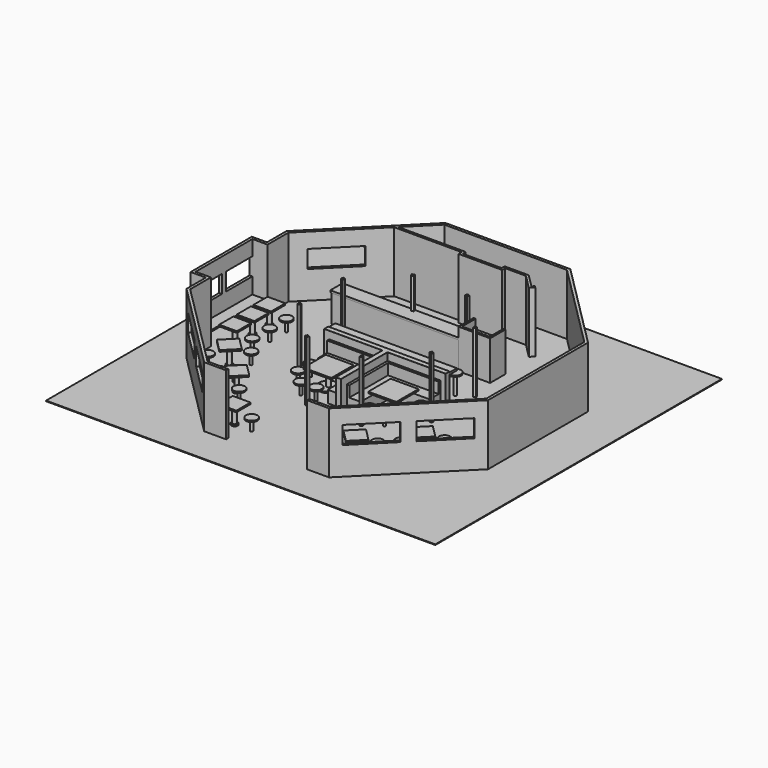
from build123d import *

# Parameters (mm, degrees)
F6_W      = 200
F6_H      = 200
F7_DEPTH  = 1200
F9_DEPTH  = 900
F11_DEPTH = 470
F13_DEPTH = 60
F15_DEPTH = 2400
F17_DEPTH = 2400
F16_W     = 110
F16_H     = 200
F19_W     = 5059.252981
F19_H     = 600
F20_DEPTH = 80
F22_DEPTH = 1550
F23_R     = 3
F25_DEPTH = 80
F27_W     = 110
F27_H     = 1300
F28_DEPTH = 600
F29_W     = 110
F29_H     = 1300
F30_DEPTH = 1100
F31_W     = 5019.252981
F31_H     = 560
F32_DEPTH = 1120
F34_DEPTH = 50
F33_R     = 225
F36_R     = 225
F37_DEPTH = 50
F38_R     = 50
F39_DEPTH = 450
F40_R     = 50
F41_DEPTH = 780
F42_R     = 125
F43_DEPTH = 50
F42_R_2   = 75
F44_R     = 75
F45_DEPTH = 680
F46_R     = 375
F47_DEPTH = 50
F48_R     = 75
F49_DEPTH = 620
F50_W     = 15369.4958686829
F50_H     = 14148.3583450317
F51_DEPTH = 25


# Not quite as in the source:
# - ends of sketch curves that miss each other by under 0.0002 mm in the source are joined


with BuildPart() as f7:
    # F6 (on offset) → F7 (new body)
    with BuildSketch(Plane.XY.offset(1200)):
        Polygon((-108.954118, -103.028913), (-108.954118, 96.971087), (-2306.968571, 96.971087), (-2408.954118, 96.971087), (-2408.954118, -103.028913), (-2208.968571, -103.028913), align=None)
        with Locations((-8.954118, -3.028913)):
            Rectangle(F6_W, F6_H)
        Polygon((91.045882, -103.028913), (-108.954118, -103.028913), (-108.954118, -2112.146564), (-108.954118, -2400), (91.045882, -2400), (91.045882, -2112.146564), align=None)
        Polygon((2289.060335, 96.971087), (91.045882, 96.971087), (91.045882, -103.028913), (2191.060335, -103.028913), (2391.045882, -103.028913), (2391.045882, 96.971087), align=None)
    extrude(amount=-F7_DEPTH)

    # F8 (on offset) → F9 (join)
    with BuildSketch(Plane.XY.offset(900)):
        Polygon((-108.954118, -2112.146564), (-108.954118, -103.028913), (-2208.968571, -103.028913), (-2208.968571, -203.028913), (-208.954118, -203.028913), (-208.954118, -2112.146564), align=None)
        Polygon((91.045882, -103.028913), (91.045882, -2112.146564), (191.045882, -2112.146564), (191.045882, -203.028913), (2191.060335, -203.028913), (2191.060335, -103.028913), align=None)
    extrude(amount=-F9_DEPTH)

    # F10 (on offset) → F11 (join)
    with BuildSketch(Plane.XY.offset(470)):
        Polygon((-2208.968571, -653.028913), (-658.954118, -653.028913), (-658.954118, -2112.146564), (-208.954118, -2112.146564), (-208.954118, -203.028913), (-2208.968571, -203.028913), align=None)
        Polygon((641.045882, -653.028913), (2191.060335, -653.028913), (2191.060335, -203.028913), (191.045882, -203.028913), (191.045882, -2112.146564), (641.045882, -2112.146564), align=None)
    extrude(amount=-F11_DEPTH)

    # F23
    f23_edges = [f7.edges().sort_by_distance(p)[0] for p in [
        (-2408.954118, -3.028913, 1200),
        (-1258.954118, -103.028913, 1200),
        (-108.954118, -1251.514457, 1200),
        (-8.954118, -2400, 1200),
        (91.045882, -1251.514457, 1200),
        (1241.045882, -103.028913, 1200),
        (2391.045882, -3.028913, 1200),
        (-8.954118, 96.971087, 1200),
        (-108.954118, -2400, 600),
        (91.045882, -2400, 600),
        (-8.954118, -2400, 0),
        (2391.045882, -103.028913, 600),
        (2391.045882, 96.971087, 600),
        (2391.045882, -3.028913, 0),
        (-2408.954118, 96.971087, 600),
        (-2408.954118, -103.028913, 600),
        (-2408.954118, -3.028913, 0),
    ]]
    fillet(f23_edges, radius=F23_R)

    # F24 (on offset) → F25 (join)
    with BuildSketch(Plane.XY.offset(1170)):
        Polygon((-2306.968571, 96.971087), (-108.954118, 96.971087), (91.045882, 96.971087), (2289.060335, 96.971087), (2391.045882, 96.971087), (2391.045882, 446.971087), (-2408.954118, 446.971087), (-2408.954118, 96.971087), align=None)
    extrude(amount=-F25_DEPTH)


with BuildPart() as f13:
    # F12 (on offset) → F13 (new body)
    with BuildSketch(Plane.XY.offset(740)):
        with BuildLine():
            ThreePointArc((-4963.658117, 1167.786273), (-4965.1225830941, 1171.3218069059), (-4968.658117, 1172.786273))
            Line((-4968.658117, 1172.786273), (-5658.658117, 1172.786273))
            ThreePointArc((-5658.658117, 1172.786273), (-5662.1936509059, 1171.3218069059), (-5663.658117, 1167.786273))
            Line((-5663.658117, 1167.786273), (-5663.658117, 477.786273))
            ThreePointArc((-5663.658117, 477.786273), (-5662.1936509059, 474.2507390941), (-5658.658117, 472.786273))
            Line((-5658.658117, 472.786273), (-4968.658117, 472.786273))
            ThreePointArc((-4968.658117, 472.786273), (-4965.1225830941, 474.2507390941), (-4963.658117, 477.786273))
            Line((-4963.658117, 477.786273), (-4963.658117, 1167.786273))
        make_face()
    extrude(amount=-F13_DEPTH)


with BuildPart() as f13b:
    # F12 (on offset) → F13, piece 2 (new body)
    with BuildSketch(Plane.XY.offset(740)):
        with BuildLine():
            ThreePointArc((-4963.658117, 345), (-4965.1225830941, 348.5355339059), (-4968.658117, 350))
            Line((-4968.658117, 350), (-5658.658117, 350))
            ThreePointArc((-5658.658117, 350), (-5662.1936509059, 348.5355339059), (-5663.658117, 345))
            Line((-5663.658117, 345), (-5663.658117, -345))
            ThreePointArc((-5663.658117, -345), (-5662.1936509059, -348.5355339059), (-5658.658117, -350))
            Line((-5658.658117, -350), (-4968.658117, -350))
            ThreePointArc((-4968.658117, -350), (-4965.1225830941, -348.5355339059), (-4963.658117, -345))
            Line((-4963.658117, -345), (-4963.658117, 345))
        make_face()
    extrude(amount=-F13_DEPTH)


with BuildPart() as f13c:
    # F12 (on offset) → F13, piece 3 (new body)
    with BuildSketch(Plane.XY.offset(740)):
        with BuildLine():
            ThreePointArc((-4963.658117, -522.261207), (-4965.1225830941, -518.7256730941), (-4968.658117, -517.261207))
            Line((-4968.658117, -517.261207), (-5658.658117, -517.261207))
            ThreePointArc((-5658.658117, -517.261207), (-5662.1936509059, -518.7256730941), (-5663.658117, -522.261207))
            Line((-5663.658117, -522.261207), (-5663.658117, -1212.261207))
            ThreePointArc((-5663.658117, -1212.261207), (-5662.1936509059, -1215.7967409059), (-5658.658117, -1217.261207))
            Line((-5658.658117, -1217.261207), (-4968.658117, -1217.261207))
            ThreePointArc((-4968.658117, -1217.261207), (-4965.1225830941, -1215.7967409059), (-4963.658117, -1212.261207))
            Line((-4963.658117, -1212.261207), (-4963.658117, -522.261207))
        make_face()
    extrude(amount=-F13_DEPTH)


with BuildPart() as f13d:
    # F12 (on offset) → F13, piece 4 (new body)
    with BuildSketch(Plane.XY.offset(740)):
        with BuildLine():
            ThreePointArc((-4594.1336350941, -1555.8954520941), (-4597.669169, -1554.430986), (-4601.2047029059, -1555.8954520941))
            Line((-4601.2047029059, -1555.8954520941), (-5089.108382, -2043.799131))
            ThreePointArc((-5089.108382, -2043.799131), (-5090.572848, -2047.334665), (-5089.1083819059, -2050.8701989059))
            Line((-5089.1083819059, -2050.8701989059), (-4601.204703, -2538.773878))
            ThreePointArc((-4601.204703, -2538.773878), (-4597.669169, -2540.238344), (-4594.1336350941, -2538.7738779059))
            Line((-4594.1336350941, -2538.7738779059), (-4106.229956, -2050.870199))
            ThreePointArc((-4106.229956, -2050.870199), (-4104.76549, -2047.334665), (-4106.2299560941, -2043.7991310941))
            Line((-4106.2299560941, -2043.7991310941), (-4594.1336350941, -1555.8954520941))
        make_face()
    extrude(amount=-F13_DEPTH)


with BuildPart() as f13e:
    # F12 (on offset) → F13, piece 5 (new body)
    with BuildSketch(Plane.XY.offset(740)):
        with BuildLine():
            ThreePointArc((-3818.2484069059, -3268.8028690941), (-3819.712873, -3272.338403), (-3818.2484069059, -3275.8739369059))
            Line((-3818.2484069059, -3275.8739369059), (-3330.344728, -3763.777616))
            ThreePointArc((-3330.344728, -3763.777616), (-3326.809194, -3765.242082), (-3323.2736600941, -3763.7776159059))
            Line((-3323.2736600941, -3763.7776159059), (-2835.369981, -3275.873937))
            ThreePointArc((-2835.369981, -3275.873937), (-2833.905515, -3272.338403), (-2835.3699810941, -3268.8028690941))
            Line((-2835.3699810941, -3268.8028690941), (-3323.27366, -2780.89919))
            ThreePointArc((-3323.27366, -2780.89919), (-3326.809194, -2779.434724), (-3330.3447279059, -2780.8991900941))
            Line((-3330.3447279059, -2780.8991900941), (-3818.2484069059, -3268.8028690941))
        make_face()
    extrude(amount=-F13_DEPTH)


with BuildPart() as f13f:
    # F12 (on offset) → F13, piece 6 (new body)
    with BuildSketch(Plane.XY.offset(740)):
        with BuildLine():
            ThreePointArc((-4356.2172039059, -3789.6932920941), (-4357.68167, -3793.228826), (-4356.2172039059, -3796.7643599059))
            Line((-4356.2172039059, -3796.7643599059), (-3868.313525, -4284.668039))
            ThreePointArc((-3868.313525, -4284.668039), (-3864.7779913536, -4286.132505), (-3861.2424575941, -4284.6680394059))
            Line((-3861.2424575941, -4284.6680394059), (-3373.338779, -3796.76436))
            ThreePointArc((-3373.338779, -3796.76436), (-3371.874312, -3793.228826), (-3373.3387785941, -3789.6932915941))
            Line((-3373.3387785941, -3789.6932915941), (-3861.242458, -3301.789613))
            ThreePointArc((-3861.242458, -3301.789613), (-3864.7779913536, -3300.325147), (-3868.3135249059, -3301.7896130941))
            Line((-3868.3135249059, -3301.7896130941), (-4356.2172039059, -3789.6932920941))
        make_face()
    extrude(amount=-F13_DEPTH)


with BuildPart() as f13g:
    # F12 (on offset) → F13, piece 7 (new body)
    with BuildSketch(Plane.XY.offset(740)):
        with BuildLine():
            Line((-2362.946575, -4675.311307), (-2362.946575, -5365.311307))
            ThreePointArc((-2362.946575, -5365.311307), (-2361.4821089059, -5368.8468409059), (-2357.946575, -5370.311307))
            Line((-2357.946575, -5370.311307), (-1667.946575, -5370.311307))
            ThreePointArc((-1667.946575, -5370.311307), (-1664.4110410941, -5368.8468409059), (-1662.946575, -5365.311307))
            Line((-1662.946575, -5365.311307), (-1662.946575, -4675.311307))
            ThreePointArc((-1662.946575, -4675.311307), (-1664.4110410941, -4671.7757730941), (-1667.946575, -4670.311307))
            Line((-1667.946575, -4670.311307), (-2357.946575, -4670.311307))
            ThreePointArc((-2357.946575, -4670.311307), (-2361.4821089059, -4671.7757730941), (-2362.946575, -4675.311307))
        make_face()
    extrude(amount=-F13_DEPTH)


with BuildPart() as f13h:
    # F12 (on offset) → F13, piece 8 (new body)
    with BuildSketch(Plane.XY.offset(740)):
        with BuildLine():
            Line((2285.312608, -4868.218593), (2773.216287, -5356.122273))
            ThreePointArc((2773.216287, -5356.122273), (2776.7518206464, -5357.586739), (2780.2873544059, -5356.1222734059))
            Line((2780.2873544059, -5356.1222734059), (3268.191034, -4868.218593))
            ThreePointArc((3268.191034, -4868.218593), (3269.6555, -4864.6830596464), (3268.1910339059, -4861.1475260941))
            Line((3268.1910339059, -4861.1475260941), (2780.287354, -4373.243847))
            ThreePointArc((2780.287354, -4373.243847), (2776.7518206464, -4371.779381), (2773.2162870941, -4373.2438470941))
            Line((2773.2162870941, -4373.2438470941), (2285.312608, -4861.147526))
            ThreePointArc((2285.312608, -4861.147526), (2283.848142, -4864.6830596464), (2285.312608, -4868.218593))
        make_face()
    extrude(amount=-F13_DEPTH)


with BuildPart() as f13i:
    # F12 (on offset) → F13, piece 9 (new body)
    with BuildSketch(Plane.XY.offset(740)):
        with BuildLine():
            Line((1747.34381, -4347.32817), (2235.247489, -4835.231849))
            ThreePointArc((2235.247489, -4835.231849), (2238.783023, -4836.696315), (2242.3185569059, -4835.2318489059))
            Line((2242.3185569059, -4835.2318489059), (2730.222236, -4347.32817))
            ThreePointArc((2730.222236, -4347.32817), (2731.686702, -4343.7926363536), (2730.2222364059, -4340.2571025941))
            Line((2730.2222364059, -4340.2571025941), (2242.318557, -3852.353424))
            ThreePointArc((2242.318557, -3852.353424), (2238.783023, -3850.888957), (2235.2474885941, -3852.3534235941))
            Line((2235.2474885941, -3852.3534235941), (1747.34381, -4340.257103))
            ThreePointArc((1747.34381, -4340.257103), (1745.879344, -4343.7926363536), (1747.34381, -4347.32817))
        make_face()
    extrude(amount=-F13_DEPTH)


with BuildPart() as f13j:
    # F12 (on offset) → F13, piece 10 (new body)
    with BuildSketch(Plane.XY.offset(740)):
        with BuildLine():
            Line((3758.322411, -3409.440769), (4246.22609, -3897.344448))
            ThreePointArc((4246.22609, -3897.344448), (4249.761624, -3898.808914), (4253.2971579059, -3897.3444479059))
            Line((4253.2971579059, -3897.3444479059), (4741.200837, -3409.440769))
            ThreePointArc((4741.200837, -3409.440769), (4742.665303, -3405.905235), (4741.2008369059, -3402.3697010941))
            Line((4741.2008369059, -3402.3697010941), (4253.297158, -2914.466022))
            ThreePointArc((4253.297158, -2914.466022), (4249.761624, -2913.001556), (4246.2260900941, -2914.4660220941))
            Line((4246.2260900941, -2914.4660220941), (3758.322411, -3402.369701))
            ThreePointArc((3758.322411, -3402.369701), (3756.857945, -3405.905235), (3758.322411, -3409.440769))
        make_face()
    extrude(amount=-F13_DEPTH)


with BuildPart() as f13k:
    # F12 (on offset) → F13, piece 11 (new body)
    with BuildSketch(Plane.XY.offset(740)):
        with BuildLine():
            ThreePointArc((721.045882, -1830.028913), (722.5103480941, -1833.5644469059), (726.045882, -1835.028913))
            Line((726.045882, -1835.028913), (1818.045882, -1835.028913))
            ThreePointArc((1818.045882, -1835.028913), (1821.5814159059, -1833.5644469059), (1823.045882, -1830.028913))
            Line((1823.045882, -1830.028913), (1823.045882, -738.028913))
            ThreePointArc((1823.045882, -738.028913), (1821.5814159059, -734.4933790941), (1818.045882, -733.028913))
            Line((1818.045882, -733.028913), (726.045882, -733.028913))
            ThreePointArc((726.045882, -733.028913), (722.5103480941, -734.4933790941), (721.045882, -738.028913))
            Line((721.045882, -738.028913), (721.045882, -1830.028913))
        make_face()
    extrude(amount=-F13_DEPTH)


with BuildPart() as f13l:
    # F12 (on offset) → F13, piece 12 (new body)
    with BuildSketch(Plane.XY.offset(740)):
        with BuildLine():
            Line((-1840.954118, -738.028913), (-1840.954118, -1830.028913))
            ThreePointArc((-1840.954118, -1830.028913), (-1839.4896519059, -1833.5644469059), (-1835.954118, -1835.028913))
            Line((-1835.954118, -1835.028913), (-743.954118, -1835.028913))
            ThreePointArc((-743.954118, -1835.028913), (-740.4185840941, -1833.5644469059), (-738.954118, -1830.028913))
            Line((-738.954118, -1830.028913), (-738.954118, -738.028913))
            ThreePointArc((-738.954118, -738.028913), (-740.4185840941, -734.4933790941), (-743.954118, -733.028913))
            Line((-743.954118, -733.028913), (-1835.954118, -733.028913))
            ThreePointArc((-1835.954118, -733.028913), (-1839.4896519059, -734.4933790941), (-1840.954118, -738.028913))
        make_face()
    extrude(amount=-F13_DEPTH)


with BuildPart() as f13m:
    # F12 (on offset) → F13, piece 13 (new body)
    with BuildSketch(Plane.XY.offset(740)):
        with BuildLine():
            Line((3220.353613, -2888.550346), (3708.257292, -3376.454025))
            ThreePointArc((3708.257292, -3376.454025), (3711.792826, -3377.918491), (3715.3283599059, -3376.4540249059))
            Line((3715.3283599059, -3376.4540249059), (4203.232039, -2888.550346))
            ThreePointArc((4203.232039, -2888.550346), (4204.696505, -2885.014812), (4203.2320389059, -2881.4792780941))
            Line((4203.2320389059, -2881.4792780941), (3715.32836, -2393.575599))
            ThreePointArc((3715.32836, -2393.575599), (3711.792826, -2392.111133), (3708.2572920941, -2393.5755990941))
            Line((3708.2572920941, -2393.5755990941), (3220.353613, -2881.479278))
            ThreePointArc((3220.353613, -2881.479278), (3218.889147, -2885.014812), (3220.353613, -2888.550346))
        make_face()
    extrude(amount=-F13_DEPTH)


with BuildPart() as f15:
    # F14 (on Top) → F15 (new body)
    with BuildSketch(Plane.XY):
        with BuildLine():
            Line((-1140.652062, 2633.066999), (-1104.679819, 2546.222323))
            ThreePointArc((-1104.679819, 2546.222323), (-1103.0562305162, 2544.5987344932), (-1100.7601297452, 2544.5987343849))
            Line((-1100.7601297452, 2544.5987343849), (-1013.915454, 2580.570977))
            ThreePointArc((-1013.915454, 2580.570977), (-1012.2918654932, 2582.1945654838), (-1012.2918653849, 2584.4906662548))
            Line((-1012.2918653849, 2584.4906662548), (-1048.264108, 2671.335342))
            ThreePointArc((-1048.264108, 2671.335342), (-1049.887696307, 2672.9589304336), (-1052.1837969012, 2672.9589307615))
            Line((-1052.1837969012, 2672.9589307615), (-1139.028473, 2636.986688))
            ThreePointArc((-1139.028473, 2636.986688), (-1140.6520614336, 2635.363099693), (-1140.652062, 2633.066999))
        make_face()
    extrude(amount=F15_DEPTH)


with BuildPart() as f15b:
    # F14 (on Top) → F15, piece 2 (new body)
    with BuildSketch(Plane.XY):
        with BuildLine():
            ThreePointArc((1012.2918653849, 2584.4906662548), (1012.2918654932, 2582.1945654838), (1013.9154540988, 2580.5709772385))
            Line((1013.9154540988, 2580.5709772385), (1100.76013, 2544.598735))
            ThreePointArc((1100.76013, 2544.598735), (1103.0562305162, 2544.5987344932), (1104.6798187615, 2546.2223230988))
            Line((1104.6798187615, 2546.2223230988), (1140.652062, 2633.066999))
            ThreePointArc((1140.652062, 2633.066999), (1140.6520614336, 2635.363099693), (1139.0284729012, 2636.9866877615))
            Line((1139.0284729012, 2636.9866877615), (1052.183797, 2672.958931))
            ThreePointArc((1052.183797, 2672.958931), (1049.887696307, 2672.9589304336), (1048.2641082385, 2671.3353419012))
            Line((1048.2641082385, 2671.3353419012), (1012.2918653849, 2584.4906662548))
        make_face()
    extrude(amount=F15_DEPTH)


with BuildPart() as f15c:
    # F14 (on Top) → F15, piece 3 (new body)
    with BuildSketch(Plane.XY):
        with BuildLine():
            ThreePointArc((-2584.4906662548, 1012.2918653849), (-2582.1945654838, 1012.2918654932), (-2580.5709772385, 1013.9154540988))
            Line((-2580.5709772385, 1013.9154540988), (-2544.598735, 1100.76013))
            ThreePointArc((-2544.598735, 1100.76013), (-2544.5987344932, 1103.0562305162), (-2546.2223230988, 1104.6798187615))
            Line((-2546.2223230988, 1104.6798187615), (-2633.066999, 1140.652062))
            ThreePointArc((-2633.066999, 1140.652062), (-2635.363099693, 1140.6520614336), (-2636.9866877615, 1139.0284729012))
            Line((-2636.9866877615, 1139.0284729012), (-2672.958931, 1052.183797))
            ThreePointArc((-2672.958931, 1052.183797), (-2672.9589304336, 1049.887696307), (-2671.3353419012, 1048.2641082385))
            Line((-2671.3353419012, 1048.2641082385), (-2584.4906662548, 1012.2918653849))
        make_face()
    extrude(amount=F15_DEPTH)


with BuildPart() as f15d:
    # F14 (on Top) → F15, piece 4 (new body)
    with BuildSketch(Plane.XY):
        with BuildLine():
            Line((-2633.066999, -1140.652062), (-2546.222323, -1104.679819))
            ThreePointArc((-2546.222323, -1104.679819), (-2544.5987344932, -1103.0562305162), (-2544.5987343849, -1100.7601297452))
            Line((-2544.5987343849, -1100.7601297452), (-2580.570977, -1013.915454))
            ThreePointArc((-2580.570977, -1013.915454), (-2582.1945654838, -1012.2918654932), (-2584.4906662548, -1012.2918653849))
            Line((-2584.4906662548, -1012.2918653849), (-2671.335342, -1048.264108))
            ThreePointArc((-2671.335342, -1048.264108), (-2672.9589304336, -1049.887696307), (-2672.9589307615, -1052.1837969012))
            Line((-2672.9589307615, -1052.1837969012), (-2636.986688, -1139.028473))
            ThreePointArc((-2636.986688, -1139.028473), (-2635.363099693, -1140.6520614336), (-2633.066999, -1140.652062))
        make_face()
    extrude(amount=F15_DEPTH)


with BuildPart() as f15e:
    # F14 (on Top) → F15, piece 5 (new body)
    with BuildSketch(Plane.XY):
        with BuildLine():
            ThreePointArc((-1012.2918653849, -2584.4906662548), (-1012.2918654932, -2582.1945654838), (-1013.9154540988, -2580.5709772385))
            Line((-1013.9154540988, -2580.5709772385), (-1100.76013, -2544.598735))
            ThreePointArc((-1100.76013, -2544.598735), (-1103.0562305162, -2544.5987344932), (-1104.6798187615, -2546.2223230988))
            Line((-1104.6798187615, -2546.2223230988), (-1140.652062, -2633.066999))
            ThreePointArc((-1140.652062, -2633.066999), (-1140.6520614336, -2635.363099693), (-1139.0284729012, -2636.9866877615))
            Line((-1139.0284729012, -2636.9866877615), (-1052.183797, -2672.958931))
            ThreePointArc((-1052.183797, -2672.958931), (-1049.887696307, -2672.9589304336), (-1048.2641082385, -2671.3353419012))
            Line((-1048.2641082385, -2671.3353419012), (-1012.2918653849, -2584.4906662548))
        make_face()
    extrude(amount=F15_DEPTH)


with BuildPart() as f15f:
    # F14 (on Top) → F15, piece 6 (new body)
    with BuildSketch(Plane.XY):
        with BuildLine():
            Line((1140.652062, -2633.066999), (1104.679819, -2546.222323))
            ThreePointArc((1104.679819, -2546.222323), (1103.0562305162, -2544.5987344932), (1100.7601297452, -2544.5987343849))
            Line((1100.7601297452, -2544.5987343849), (1013.915454, -2580.570977))
            ThreePointArc((1013.915454, -2580.570977), (1012.2918654932, -2582.1945654838), (1012.2918653849, -2584.4906662548))
            Line((1012.2918653849, -2584.4906662548), (1048.264108, -2671.335342))
            ThreePointArc((1048.264108, -2671.335342), (1049.887696307, -2672.9589304336), (1052.1837969012, -2672.9589307615))
            Line((1052.1837969012, -2672.9589307615), (1139.028473, -2636.986688))
            ThreePointArc((1139.028473, -2636.986688), (1140.6520614336, -2635.363099693), (1140.652062, -2633.066999))
        make_face()
    extrude(amount=F15_DEPTH)


with BuildPart() as f15g:
    # F14 (on Top) → F15, piece 7 (new body)
    with BuildSketch(Plane.XY):
        with BuildLine():
            ThreePointArc((2584.4906662548, -1012.2918653849), (2582.1945654838, -1012.2918654932), (2580.5709772385, -1013.9154540988))
            Line((2580.5709772385, -1013.9154540988), (2544.598735, -1100.76013))
            ThreePointArc((2544.598735, -1100.76013), (2544.5987344932, -1103.0562305162), (2546.2223230988, -1104.6798187615))
            Line((2546.2223230988, -1104.6798187615), (2633.066999, -1140.652062))
            ThreePointArc((2633.066999, -1140.652062), (2635.363099693, -1140.6520614336), (2636.9866877615, -1139.0284729012))
            Line((2636.9866877615, -1139.0284729012), (2672.958931, -1052.183797))
            ThreePointArc((2672.958931, -1052.183797), (2672.9589304336, -1049.887696307), (2671.3353419012, -1048.2641082385))
            Line((2671.3353419012, -1048.2641082385), (2584.4906662548, -1012.2918653849))
        make_face()
    extrude(amount=F15_DEPTH)


with BuildPart() as f15h:
    # F14 (on Top) → F15, piece 8 (new body)
    with BuildSketch(Plane.XY):
        with BuildLine():
            Line((2633.066999, 1140.652062), (2546.222323, 1104.679819))
            ThreePointArc((2546.222323, 1104.679819), (2544.5987344932, 1103.0562305162), (2544.5987343849, 1100.7601297452))
            Line((2544.5987343849, 1100.7601297452), (2580.570977, 1013.915454))
            ThreePointArc((2580.570977, 1013.915454), (2582.1945654838, 1012.2918654932), (2584.4906662548, 1012.2918653849))
            Line((2584.4906662548, 1012.2918653849), (2671.335342, 1048.264108))
            ThreePointArc((2671.335342, 1048.264108), (2672.9589304336, 1049.887696307), (2672.9589307615, 1052.1837969012))
            Line((2672.9589307615, 1052.1837969012), (2636.986688, 1139.028473))
            ThreePointArc((2636.986688, 1139.028473), (2635.363099693, 1140.6520614336), (2633.066999, 1140.652062))
        make_face()
    extrude(amount=F15_DEPTH)


with BuildPart() as f17:
    # F16 (on Top) → F17 (new body)
    with BuildSketch(Plane.XY):
        Polygon((-2466.641764, 5955), (-4225.725471, 4195.916293), (-4147.943725, 4118.134547), (-3521.078272, 4745), (-860, 4745), (-860, 4595), (860, 4595), (860, 4745), (1682.600641, 4745), (2248.286066, 4179.314575), (2389.707422, 4320.735931), (2326.067812, 4384.375542), (2248.286066, 4306.593796), (1719.879862, 4835), (770, 4835), (770, 4685), (-770, 4685), (-770, 4835), (-3431.078272, 4835), (-2421.078272, 5845), align=None)
        Polygon((2466.641764, 5955), (-2466.641764, 5955), (-2421.078272, 5845), (2421.078272, 5845), (4757.132034, 3508.946238), (5845, 2421.078272), (5955, 2466.641764), align=None)
        Polygon((5955, -2466.641764), (5955, 2466.641764), (5845, 2421.078272), (5845, -2421.078272), (5582.608037, -2683.470235), (5660.389783, -2761.251981), align=None)
    extrude(amount=F17_DEPTH)



with BuildPart() as f17b:
    # F16 (on Top) → F17, piece 2 (new body)
    with BuildSketch(Plane.XY):
        Polygon((-5922.781746, 2498.860018), (-5845, 2421.078272), (-5420.735931, 2845.342341), (-5498.517677, 2923.124087), align=None)
        Polygon((-5845, 1400), (-5845, 2421.078272), (-5922.781746, 2498.860018), (-5955, 2466.641764), (-5955, 1510), (-6555, 1510), (-6555, 1400), (-6445, 1400), (-5955, 1400), align=None)
    extrude(amount=F17_DEPTH)


with BuildPart() as f17c:
    # F16 (on Top) → F17, piece 3 (new body)
    with BuildSketch(Plane.XY):
        with Locations((-6500, 0)):
            Rectangle(F16_W, F16_H)
    extrude(amount=F17_DEPTH)


with BuildPart() as f17d:
    # F16 (on Top) → F17, piece 4 (new body)
    with BuildSketch(Plane.XY):
        Polygon((-6555, -1510), (-5955, -1510), (-5955, -2466.641764), (-5660.389783, -2761.251981), (-5582.608037, -2683.470235), (-5845, -2421.078272), (-5845, -1400), (-5955, -1400), (-6445, -1400), (-6555, -1400), align=None)
    extrude(amount=F17_DEPTH)


with BuildPart() as f17e:
    # F16 (on Top) → F17, piece 5 (new body)
    with BuildSketch(Plane.XY):
        Polygon((-3956.262441, -4309.815831), (-4309.815831, -3956.262441), (-4387.597577, -4034.044187), (-4034.044187, -4387.597577), align=None)
    extrude(amount=F17_DEPTH)


with BuildPart() as f17f:
    # F16 (on Top) → F17, piece 6 (new body)
    with BuildSketch(Plane.XY):
        Polygon((-2466.641764, -5955), (-1600, -5955), (-1600, -5845), (-2421.078272, -5845), (-2683.470235, -5582.608037), (-2761.251981, -5660.389783), align=None)
    extrude(amount=F17_DEPTH)


with BuildPart() as f17g:
    # F16 (on Top) → F17, piece 7 (new body)
    with BuildSketch(Plane.XY):
        Polygon((2683.470235, -5582.608037), (2421.078272, -5845), (1600, -5845), (1600, -5955), (2466.641764, -5955), (2761.251981, -5660.389783), align=None)
    extrude(amount=F17_DEPTH)


with BuildPart() as f17h:
    # F16 (on Top) → F17, piece 8 (new body)
    with BuildSketch(Plane.XY):
        Polygon((4309.815831, -3956.262441), (3956.262441, -4309.815831), (4034.044187, -4387.597577), (4387.597577, -4034.044187), align=None)
    extrude(amount=F17_DEPTH)


with BuildPart() as f20:
    # F19 (on offset) → F20 (new body)
    with BuildSketch(Plane.XY.offset(1170)):
        with Locations((-1375.3735095, 2373.450684)):
            Rectangle(F19_W, F19_H)
    extrude(amount=-F20_DEPTH)

    # F21 (on offset) → F22 (join)
    with BuildSketch(Plane.XY.offset(1550)):
        Polygon((1154.252981, 2823.450684), (1154.252981, 2673.450684), (1154.252981, 2073.450684), (2404.252981, 2073.450684), (2404.252981, 2823.450684), (2324.252981, 2823.450684), (2324.252981, 2153.450684), (1234.252981, 2153.450684), (1234.252981, 2823.450684), align=None)
    extrude(amount=-F22_DEPTH)


with BuildPart() as f17_1:
    add(f17.part)

    add(f17b.part)  # F28 merges F17b

    add(f17c.part)  # F28 merges F17c

    add(f17d.part)  # F28 merges F17d

    add(f17e.part)  # F28 merges F17e

    add(f17f.part)  # F28 merges F17f

    add(f17g.part)  # F28 merges F17g

    add(f17h.part)  # F28 merges F17h
    # F27 (on offset) → F28 (join)
    with BuildSketch(Plane.XY.offset(2400)):
        Polygon((-5498.517677, 2923.124087), (-5420.735931, 2845.342341), (-4147.943725, 4118.134547), (-4225.725471, 4195.916293), align=None)
        with Locations((-6500, 750)):
            Rectangle(F27_W, F27_H)
        Polygon((-4309.815831, -3956.262441), (-5582.608037, -2683.470235), (-5660.389783, -2761.251981), (-4387.597577, -4034.044187), align=None)
        Polygon((-4034.044187, -4387.597577), (-2761.251981, -5660.389783), (-2683.470235, -5582.608037), (-3956.262441, -4309.815831), align=None)
        Polygon((4034.044187, -4387.597577), (3956.262441, -4309.815831), (2683.470235, -5582.608037), (2761.251981, -5660.389783), align=None)
        Polygon((5582.608037, -2683.470235), (5322.817459, -2943.260813), (4309.815831, -3956.262441), (4387.597577, -4034.044187), (5660.389783, -2761.251981), align=None)
        with Locations((-6500, -750)):
            Rectangle(F27_W, F27_H)
    extrude(amount=-F28_DEPTH)

    # F29 (on Top) → F30 (join)
    with BuildSketch(Plane.XY):
        Polygon((5582.608037, -2683.470235), (5322.817459, -2943.260813), (4309.815831, -3956.262441), (4387.597577, -4034.044187), (5660.389783, -2761.251981), align=None)
        Polygon((4034.044187, -4387.597577), (3956.262441, -4309.815831), (2683.470235, -5582.608037), (2761.251981, -5660.389783), align=None)
        Polygon((-4309.815831, -3956.262441), (-5582.608037, -2683.470235), (-5660.389783, -2761.251981), (-4387.597577, -4034.044187), align=None)
        Polygon((-4034.044187, -4387.597577), (-2761.251981, -5660.389783), (-2683.470235, -5582.608037), (-3956.262441, -4309.815831), align=None)
        with Locations((-6500, -750)):
            Rectangle(F29_W, F29_H)
        with Locations((-6500, 750)):
            Rectangle(F29_W, F29_H)
        Polygon((-5498.517677, 2923.124087), (-5420.735931, 2845.342341), (-4147.943725, 4118.134547), (-4225.725471, 4195.916293), align=None)
    extrude(amount=F30_DEPTH)

    # F33 (on offset) → F34 (join)
    with BuildSketch(Plane.XY.offset(470)):
        with BuildLine():
            ThreePointArc((-5955, -120.3832677743), (-6113.658117, 0), (-5955, 120.3832677743))
            Line((-5955, 120.3832677743), (-5955, 702.4030052257))
            ThreePointArc((-5955, 702.4030052257), (-6113.658117, 822.786273), (-5955, 943.1695407743))
            Line((-5955, 943.1695407743), (-5955, 1400))
            Line((-5955, 1400), (-6445, 1400))
            Line((-6445, 1400), (-6445, 100))
            Line((-6445, 100), (-6445, -100))
            Line((-6445, -100), (-6445, -1400))
            Line((-6445, -1400), (-5955, -1400))
            Line((-5955, -1400), (-5955, -987.6444747743))
            ThreePointArc((-5955, -987.6444747743), (-6113.658117, -867.261207), (-5955, -746.8779392257))
            Line((-5955, -746.8779392257), (-5955, -120.3832677743))
        make_face()
        with BuildLine():
            Line((-5955, -120.3832677743), (-5955, 120.3832677743))
            ThreePointArc((-5955, 120.3832677743), (-6113.658117, 0), (-5955, -120.3832677743))
        make_face()
        with BuildLine():
            ThreePointArc((-5955, 943.1695407743), (-6113.658117, 822.786273), (-5955, 702.4030052257))
            Line((-5955, 702.4030052257), (-5955, 943.1695407743))
        make_face()
        with BuildLine():
            Line((-5955, -987.6444747743), (-5955, -746.8779392257))
            ThreePointArc((-5955, -746.8779392257), (-6113.658117, -867.261207), (-5955, -987.6444747743))
        make_face()
    extrude(amount=-F34_DEPTH)


with BuildPart() as f32:
    # F31 (on Top) → F32 (new body)
    with BuildSketch(Plane.XY):
        with Locations((-1375.3735095, 2373.450684)):
            Rectangle(F31_W, F31_H)
    extrude(amount=F32_DEPTH)


with BuildPart() as f34:
    # F33 (on offset) → F34, piece 2 (new body)
    with BuildSketch(Plane.XY.offset(470)):
        with Locations((-5074.966247, -2524.631742)):
            Circle(F33_R)
    extrude(amount=-F34_DEPTH)


with BuildPart() as f34b:
    # F33 (on offset) → F34, piece 3 (new body)
    with BuildSketch(Plane.XY.offset(470)):
        with Locations((-4120.372092, -1570.037587)):
            Circle(F33_R)
    extrude(amount=-F34_DEPTH)


with BuildPart() as f34c:
    # F33 (on offset) → F34, piece 4 (new body)
    with BuildSketch(Plane.XY.offset(470)):
        with Locations((-4638.658117, -867.261207)):
            Circle(F33_R)
    extrude(amount=-F34_DEPTH)


with BuildPart() as f34d:
    # F33 (on offset) → F34, piece 5 (new body)
    with BuildSketch(Plane.XY.offset(470)):
        with Locations((-4638.658117, 0)):
            Circle(F33_R)
    extrude(amount=-F34_DEPTH)


with BuildPart() as f34e:
    # F33 (on offset) → F34, piece 6 (new body)
    with BuildSketch(Plane.XY.offset(470)):
        with Locations((-4638.658117, 822.786273)):
            Circle(F33_R)
    extrude(amount=-F34_DEPTH)


with BuildPart() as f34f:
    # F33 (on offset) → F34, piece 7 (new body)
    with BuildSketch(Plane.XY.offset(470)):
        with Locations((-4342.075069, -3315.931749)):
            Circle(F33_R)
    extrude(amount=-F34_DEPTH)


with BuildPart() as f34g:
    # F33 (on offset) → F34, piece 8 (new body)
    with BuildSketch(Plane.XY.offset(470)):
        with Locations((-3804.106271, -2795.041326)):
            Circle(F33_R)
    extrude(amount=-F34_DEPTH)


with BuildPart() as f34h:
    # F33 (on offset) → F34, piece 9 (new body)
    with BuildSketch(Plane.XY.offset(470)):
        with Locations((-2849.512116, -3749.63548)):
            Circle(F33_R)
    extrude(amount=-F34_DEPTH)


with BuildPart() as f34i:
    # F33 (on offset) → F34, piece 10 (new body)
    with BuildSketch(Plane.XY.offset(470)):
        with Locations((-3387.480914, -4270.525903)):
            Circle(F33_R)
    extrude(amount=-F34_DEPTH)


with BuildPart() as f34j:
    # F33 (on offset) → F34, piece 11 (new body)
    with BuildSketch(Plane.XY.offset(470)):
        with Locations((-2687.946575, -5020.311307)):
            Circle(F33_R)
    extrude(amount=-F34_DEPTH)


with BuildPart() as f34k:
    # F33 (on offset) → F34, piece 12 (new body)
    with BuildSketch(Plane.XY.offset(470)):
        with Locations((-1337.946575, -5020.311307)):
            Circle(F33_R)
    extrude(amount=-F34_DEPTH)


with BuildPart() as f34l:
    # F33 (on offset) → F34, piece 13 (new body)
    with BuildSketch(Plane.XY.offset(470)):
        with Locations((-1058.954118, -2186.501213)):
            Circle(F33_R)
    extrude(amount=-F34_DEPTH)


with BuildPart() as f34m:
    # F33 (on offset) → F34, piece 14 (new body)
    with BuildSketch(Plane.XY.offset(470)):
        with Locations((-1658.954118, -2186.501213)):
            Circle(F33_R)
    extrude(amount=-F34_DEPTH)


with BuildPart() as f34n:
    # F33 (on offset) → F34, piece 15 (new body)
    with BuildSketch(Plane.XY.offset(470)):
        with Locations((-2192.426419, -1653.028913)):
            Circle(F33_R)
    extrude(amount=-F34_DEPTH)


with BuildPart() as f34o:
    # F33 (on offset) → F34, piece 16 (new body)
    with BuildSketch(Plane.XY.offset(470)):
        with Locations((-2192.426419, -1053.028913)):
            Circle(F33_R)
    extrude(amount=-F34_DEPTH)


with BuildPart() as f34p:
    # F33 (on offset) → F34, piece 17 (new body)
    with BuildSketch(Plane.XY.offset(470)):
        with Locations((2174.518183, -1053.028913)):
            Circle(F33_R)
    extrude(amount=-F34_DEPTH)


with BuildPart() as f34q:
    # F33 (on offset) → F34, piece 18 (new body)
    with BuildSketch(Plane.XY.offset(470)):
        with Locations((2174.518183, -1653.028913)):
            Circle(F33_R)
    extrude(amount=-F34_DEPTH)


with BuildPart() as f34r:
    # F33 (on offset) → F34, piece 19 (new body)
    with BuildSketch(Plane.XY.offset(470)):
        with Locations((1041.045882, -2186.501213)):
            Circle(F33_R)
    extrude(amount=-F34_DEPTH)


with BuildPart() as f34s:
    # F33 (on offset) → F34, piece 20 (new body)
    with BuildSketch(Plane.XY.offset(470)):
        with Locations((1641.045882, -2186.501213)):
            Circle(F33_R)
    extrude(amount=-F34_DEPTH)


with BuildPart() as f34t:
    # F33 (on offset) → F34, piece 21 (new body)
    with BuildSketch(Plane.XY.offset(470)):
        with Locations((2299.454743, -5341.980137)):
            Circle(F33_R)
    extrude(amount=-F34_DEPTH)


with BuildPart() as f34u:
    # F33 (on offset) → F34, piece 22 (new body)
    with BuildSketch(Plane.XY.offset(470)):
        with Locations((1761.485946, -4821.089714)):
            Circle(F33_R)
    extrude(amount=-F34_DEPTH)


with BuildPart() as f34v:
    # F33 (on offset) → F34, piece 23 (new body)
    with BuildSketch(Plane.XY.offset(470)):
        with Locations((3254.048898, -4387.385982)):
            Circle(F33_R)
    extrude(amount=-F34_DEPTH)


with BuildPart() as f34w:
    # F33 (on offset) → F34, piece 24 (new body)
    with BuildSketch(Plane.XY.offset(470)):
        with Locations((2716.0801, -3866.495559)):
            Circle(F33_R)
    extrude(amount=-F34_DEPTH)


with BuildPart() as f34x:
    # F33 (on offset) → F34, piece 25 (new body)
    with BuildSketch(Plane.XY.offset(470)):
        with Locations((3234.495749, -3362.311889)):
            Circle(F33_R)
    extrude(amount=-F34_DEPTH)


with BuildPart() as f34y:
    # F33 (on offset) → F34, piece 26 (new body)
    with BuildSketch(Plane.XY.offset(470)):
        with Locations((3772.464546, -3883.202313)):
            Circle(F33_R)
    extrude(amount=-F34_DEPTH)


with BuildPart() as f34z:
    # F33 (on offset) → F34, piece 27 (new body)
    with BuildSketch(Plane.XY.offset(470)):
        with Locations((4727.058701, -2928.608158)):
            Circle(F33_R)
    extrude(amount=-F34_DEPTH)


with BuildPart() as f34ba:
    # F33 (on offset) → F34, piece 28 (new body)
    with BuildSketch(Plane.XY.offset(470)):
        with Locations((4189.089903, -2407.717735)):
            Circle(F33_R)
    extrude(amount=-F34_DEPTH)


with BuildPart() as f37:
    # F36 (on offset) → F37 (new body)
    with BuildSketch(Plane.XY.offset(800)):
        with Locations((-2099.351624, 763.711185)):
            Circle(F36_R)
    extrude(amount=-F37_DEPTH)


with BuildPart() as f37b:
    # F36 (on offset) → F37, piece 2 (new body)
    with BuildSketch(Plane.XY.offset(800)):
        with Locations((-1416.216643, 763.711185)):
            Circle(F36_R)
    extrude(amount=-F37_DEPTH)


with BuildPart() as f37c:
    # F36 (on offset) → F37, piece 3 (new body)
    with BuildSketch(Plane.XY.offset(800)):
        with Locations((-718.849683, 763.711185)):
            Circle(F36_R)
    extrude(amount=-F37_DEPTH)


with BuildPart() as f37d:
    # F36 (on offset) → F37, piece 4 (new body)
    with BuildSketch(Plane.XY.offset(800)):
        with Locations((6.981234, 763.711185)):
            Circle(F36_R)
    extrude(amount=-F37_DEPTH)


with BuildPart() as f37e:
    # F36 (on offset) → F37, piece 5 (new body)
    with BuildSketch(Plane.XY.offset(800)):
        with Locations((692.962611, 763.711185)):
            Circle(F36_R)
    extrude(amount=-F37_DEPTH)


with BuildPart() as f37f:
    # F36 (on offset) → F37, piece 6 (new body)
    with BuildSketch(Plane.XY.offset(800)):
        with Locations((1398.868759, 763.711185)):
            Circle(F36_R)
    extrude(amount=-F37_DEPTH)


with BuildPart() as f37g:
    # F36 (on offset) → F37, piece 7 (new body)
    with BuildSketch(Plane.XY.offset(800)):
        with Locations((2079.157344, 763.711185)):
            Circle(F36_R)
    extrude(amount=-F37_DEPTH)


with BuildPart() as f39:
    # F38 (on Top) → F39 (new body)
    with BuildSketch(Plane.XY):
        with Locations((-4638.658117, 822.786273)):
            Circle(F38_R)
    extrude(amount=F39_DEPTH)


with BuildPart() as f39b:
    # F38 (on Top) → F39, piece 2 (new body)
    with BuildSketch(Plane.XY):
        with Locations((-4638.658117, 0)):
            Circle(F38_R)
    extrude(amount=F39_DEPTH)


with BuildPart() as f39c:
    # F38 (on Top) → F39, piece 3 (new body)
    with BuildSketch(Plane.XY):
        with Locations((-4638.658117, -867.261207)):
            Circle(F38_R)
    extrude(amount=F39_DEPTH)


with BuildPart() as f39d:
    # F38 (on Top) → F39, piece 4 (new body)
    with BuildSketch(Plane.XY):
        with Locations((-4120.372092, -1570.037587)):
            Circle(F38_R)
    extrude(amount=F39_DEPTH)


with BuildPart() as f39e:
    # F38 (on Top) → F39, piece 5 (new body)
    with BuildSketch(Plane.XY):
        with Locations((-5074.966247, -2524.631742)):
            Circle(F38_R)
    extrude(amount=F39_DEPTH)


with BuildPart() as f39f:
    # F38 (on Top) → F39, piece 6 (new body)
    with BuildSketch(Plane.XY):
        with Locations((-4342.075069, -3315.931749)):
            Circle(F38_R)
    extrude(amount=F39_DEPTH)


with BuildPart() as f39g:
    # F38 (on Top) → F39, piece 7 (new body)
    with BuildSketch(Plane.XY):
        with Locations((-3804.106271, -2795.041326)):
            Circle(F38_R)
    extrude(amount=F39_DEPTH)


with BuildPart() as f39h:
    # F38 (on Top) → F39, piece 8 (new body)
    with BuildSketch(Plane.XY):
        with Locations((-3387.480914, -4270.525903)):
            Circle(F38_R)
    extrude(amount=F39_DEPTH)


with BuildPart() as f39i:
    # F38 (on Top) → F39, piece 9 (new body)
    with BuildSketch(Plane.XY):
        with Locations((-2849.512116, -3749.63548)):
            Circle(F38_R)
    extrude(amount=F39_DEPTH)


with BuildPart() as f39j:
    # F38 (on Top) → F39, piece 10 (new body)
    with BuildSketch(Plane.XY):
        with Locations((-2687.946575, -5020.311307)):
            Circle(F38_R)
    extrude(amount=F39_DEPTH)


with BuildPart() as f39k:
    # F38 (on Top) → F39, piece 11 (new body)
    with BuildSketch(Plane.XY):
        with Locations((-1337.946575, -5020.311307)):
            Circle(F38_R)
    extrude(amount=F39_DEPTH)


with BuildPart() as f39l:
    # F38 (on Top) → F39, piece 12 (new body)
    with BuildSketch(Plane.XY):
        with Locations((-2192.426419, -1053.028913)):
            Circle(F38_R)
    extrude(amount=F39_DEPTH)


with BuildPart() as f39m:
    # F38 (on Top) → F39, piece 13 (new body)
    with BuildSketch(Plane.XY):
        with Locations((-2192.426419, -1653.028913)):
            Circle(F38_R)
    extrude(amount=F39_DEPTH)


with BuildPart() as f39n:
    # F38 (on Top) → F39, piece 14 (new body)
    with BuildSketch(Plane.XY):
        with Locations((-1658.954118, -2186.501213)):
            Circle(F38_R)
    extrude(amount=F39_DEPTH)


with BuildPart() as f39o:
    # F38 (on Top) → F39, piece 15 (new body)
    with BuildSketch(Plane.XY):
        with Locations((-1058.954118, -2186.501213)):
            Circle(F38_R)
    extrude(amount=F39_DEPTH)


with BuildPart() as f39p:
    # F38 (on Top) → F39, piece 16 (new body)
    with BuildSketch(Plane.XY):
        with Locations((1041.045882, -2186.501213)):
            Circle(F38_R)
    extrude(amount=F39_DEPTH)


with BuildPart() as f39q:
    # F38 (on Top) → F39, piece 17 (new body)
    with BuildSketch(Plane.XY):
        with Locations((1641.045882, -2186.501213)):
            Circle(F38_R)
    extrude(amount=F39_DEPTH)


with BuildPart() as f39r:
    # F38 (on Top) → F39, piece 18 (new body)
    with BuildSketch(Plane.XY):
        with Locations((2174.518183, -1653.028913)):
            Circle(F38_R)
    extrude(amount=F39_DEPTH)


with BuildPart() as f39s:
    # F38 (on Top) → F39, piece 19 (new body)
    with BuildSketch(Plane.XY):
        with Locations((2174.518183, -1053.028913)):
            Circle(F38_R)
    extrude(amount=F39_DEPTH)


with BuildPart() as f39t:
    # F38 (on Top) → F39, piece 20 (new body)
    with BuildSketch(Plane.XY):
        with Locations((1761.485946, -4821.089714)):
            Circle(F38_R)
    extrude(amount=F39_DEPTH)


with BuildPart() as f39u:
    # F38 (on Top) → F39, piece 21 (new body)
    with BuildSketch(Plane.XY):
        with Locations((2299.454743, -5341.980137)):
            Circle(F38_R)
    extrude(amount=F39_DEPTH)


with BuildPart() as f39v:
    # F38 (on Top) → F39, piece 22 (new body)
    with BuildSketch(Plane.XY):
        with Locations((2716.0801, -3866.495559)):
            Circle(F38_R)
    extrude(amount=F39_DEPTH)


with BuildPart() as f39w:
    # F38 (on Top) → F39, piece 23 (new body)
    with BuildSketch(Plane.XY):
        with Locations((3254.048898, -4387.385982)):
            Circle(F38_R)
    extrude(amount=F39_DEPTH)


with BuildPart() as f39x:
    # F38 (on Top) → F39, piece 24 (new body)
    with BuildSketch(Plane.XY):
        with Locations((3234.495749, -3362.311889)):
            Circle(F38_R)
    extrude(amount=F39_DEPTH)


with BuildPart() as f39y:
    # F38 (on Top) → F39, piece 25 (new body)
    with BuildSketch(Plane.XY):
        with Locations((4189.089903, -2407.717735)):
            Circle(F38_R)
    extrude(amount=F39_DEPTH)


with BuildPart() as f39z:
    # F38 (on Top) → F39, piece 26 (new body)
    with BuildSketch(Plane.XY):
        with Locations((4727.058701, -2928.608158)):
            Circle(F38_R)
    extrude(amount=F39_DEPTH)


with BuildPart() as f39ba:
    # F38 (on Top) → F39, piece 27 (new body)
    with BuildSketch(Plane.XY):
        with Locations((3772.464546, -3883.202313)):
            Circle(F38_R)
    extrude(amount=F39_DEPTH)


with BuildPart() as f41:
    # F40 (on Top) → F41 (new body)
    with BuildSketch(Plane.XY):
        with Locations((-2099.351624, 763.711185)):
            Circle(F40_R)
    extrude(amount=F41_DEPTH)


with BuildPart() as f41b:
    # F40 (on Top) → F41, piece 2 (new body)
    with BuildSketch(Plane.XY):
        with Locations((-1416.216643, 763.711185)):
            Circle(F40_R)
    extrude(amount=F41_DEPTH)


with BuildPart() as f41c:
    # F40 (on Top) → F41, piece 3 (new body)
    with BuildSketch(Plane.XY):
        with Locations((-718.849683, 763.711185)):
            Circle(F40_R)
    extrude(amount=F41_DEPTH)


with BuildPart() as f41d:
    # F40 (on Top) → F41, piece 4 (new body)
    with BuildSketch(Plane.XY):
        with Locations((6.981234, 763.711185)):
            Circle(F40_R)
    extrude(amount=F41_DEPTH)


with BuildPart() as f41e:
    # F40 (on Top) → F41, piece 5 (new body)
    with BuildSketch(Plane.XY):
        with Locations((692.962611, 763.711185)):
            Circle(F40_R)
    extrude(amount=F41_DEPTH)


with BuildPart() as f41f:
    # F40 (on Top) → F41, piece 6 (new body)
    with BuildSketch(Plane.XY):
        with Locations((1398.868759, 763.711185)):
            Circle(F40_R)
    extrude(amount=F41_DEPTH)


with BuildPart() as f41g:
    # F40 (on Top) → F41, piece 7 (new body)
    with BuildSketch(Plane.XY):
        with Locations((2079.157344, 763.711185)):
            Circle(F40_R)
    extrude(amount=F41_DEPTH)


with BuildPart() as f43:
    # F42 (on Top) → F43 (new body)
    with BuildSketch(Plane.XY):
        with Locations((-2012.946575, -5020.311307)):
            Circle(F42_R)
    extrude(amount=F43_DEPTH)


with BuildPart() as f43b:
    # F42 (on Top) → F43, piece 2 (new body)
    with BuildSketch(Plane.XY):
        with Locations((-3864.777991, -3793.228826)):
            Circle(F42_R)
    extrude(amount=F43_DEPTH)


with BuildPart() as f43c:
    # F42 (on Top) → F43, piece 3 (new body)
    with BuildSketch(Plane.XY):
        with Locations((-3326.809194, -3272.338403)):
            Circle(F42_R)
    extrude(amount=F43_DEPTH)


with BuildPart() as f43d:
    # F42 (on Top) → F43, piece 4 (new body)
    with BuildSketch(Plane.XY):
        with Locations((-4597.669169, -2047.334665)):
            Circle(F42_R)
    extrude(amount=F43_DEPTH)


with BuildPart() as f43e:
    # F42 (on Top) → F43, piece 5 (new body)
    with BuildSketch(Plane.XY):
        with Locations((-5313.658117, -867.261207)):
            Circle(F42_R)
    extrude(amount=F43_DEPTH)


with BuildPart() as f43f:
    # F42 (on Top) → F43, piece 6 (new body)
    with BuildSketch(Plane.XY):
        with Locations((-5313.658117, 0)):
            Circle(F42_R)
        with Locations((-5313.658117, 0)):
            Circle(F42_R_2, mode=Mode.SUBTRACT)
    extrude(amount=F43_DEPTH)


with BuildPart() as f43g:
    # F42 (on Top) → F43, piece 7 (new body)
    with BuildSketch(Plane.XY):
        with Locations((-5313.658117, 822.786273)):
            Circle(F42_R)
    extrude(amount=F43_DEPTH)


with BuildPart() as f43h:
    # F42 (on Top) → F43, piece 8 (new body)
    with BuildSketch(Plane.XY):
        with Locations((2238.783023, -4343.792636)):
            Circle(F42_R)
    extrude(amount=F43_DEPTH)


with BuildPart() as f43i:
    # F42 (on Top) → F43, piece 9 (new body)
    with BuildSketch(Plane.XY):
        with Locations((2776.751821, -4864.68306)):
            Circle(F42_R)
    extrude(amount=F43_DEPTH)


with BuildPart() as f43j:
    # F42 (on Top) → F43, piece 10 (new body)
    with BuildSketch(Plane.XY):
        with Locations((3711.792826, -2885.014812)):
            Circle(F42_R)
    extrude(amount=F43_DEPTH)


with BuildPart() as f43k:
    # F42 (on Top) → F43, piece 11 (new body)
    with BuildSketch(Plane.XY):
        with Locations((4249.761624, -3405.905235)):
            Circle(F42_R)
    extrude(amount=F43_DEPTH)


with BuildPart() as f45:
    # F44 (on face) → F45 (new body)
    with BuildSketch(Plane.XY.offset(50)):
        with Locations((2238.783023, -4343.792636)):
            Circle(F44_R)
    extrude(amount=F45_DEPTH)


with BuildPart() as f45b:
    # F44 (on face) → F45, piece 2 (new body)
    with BuildSketch(Plane.XY.offset(50)):
        with Locations((2776.751821, -4864.68306)):
            Circle(F44_R)
    extrude(amount=F45_DEPTH)


with BuildPart() as f45c:
    # F44 (on face) → F45, piece 3 (new body)
    with BuildSketch(Plane.XY.offset(50)):
        with Locations((3711.792826, -2885.014812)):
            Circle(F44_R)
    extrude(amount=F45_DEPTH)


with BuildPart() as f45d:
    # F44 (on face) → F45, piece 4 (new body)
    with BuildSketch(Plane.XY.offset(50)):
        with Locations((4249.761624, -3405.905235)):
            Circle(F44_R)
    extrude(amount=F45_DEPTH)


with BuildPart() as f45e:
    # F44 (on face) → F45, piece 5 (new body)
    with BuildSketch(Plane.XY.offset(50)):
        with Locations((-2012.946575, -5020.311307)):
            Circle(F44_R)
    extrude(amount=F45_DEPTH)


with BuildPart() as f45f:
    # F44 (on face) → F45, piece 6 (new body)
    with BuildSketch(Plane.XY.offset(50)):
        with Locations((-3864.777991, -3793.228826)):
            Circle(F44_R)
    extrude(amount=F45_DEPTH)


with BuildPart() as f45g:
    # F44 (on face) → F45, piece 7 (new body)
    with BuildSketch(Plane.XY.offset(50)):
        with Locations((-3326.809194, -3272.338403)):
            Circle(F44_R)
    extrude(amount=F45_DEPTH)


with BuildPart() as f45h:
    # F44 (on face) → F45, piece 8 (new body)
    with BuildSketch(Plane.XY.offset(50)):
        with Locations((-4597.669169, -2047.334665)):
            Circle(F44_R)
    extrude(amount=F45_DEPTH)


with BuildPart() as f45i:
    # F44 (on face) → F45, piece 9 (new body)
    with BuildSketch(Plane.XY.offset(50)):
        with Locations((-5313.658117, -867.261207)):
            Circle(F44_R)
    extrude(amount=F45_DEPTH)


with BuildPart() as f45j:
    # F44 (on face) → F45, piece 10 (new body)
    with BuildSketch(Plane.XY.offset(50)):
        with Locations((-5313.658117, 822.786273)):
            Circle(F44_R)
    extrude(amount=F45_DEPTH)


with BuildPart() as f45k:
    # F44 (on face) → F45, piece 11 (new body)
    with BuildSketch(Plane.XY.offset(50)):
        with Locations((-5313.658117, 0)):
            Circle(F44_R)
    extrude(amount=F45_DEPTH)


with BuildPart() as f47:
    # F46 (on face) → F47 (new body)
    with BuildSketch(Plane.XY):
        with Locations((-1289.954118, -1284.028913)):
            Circle(F46_R)
    extrude(amount=F47_DEPTH)


with BuildPart() as f47b:
    # F46 (on face) → F47, piece 2 (new body)
    with BuildSketch(Plane.XY):
        with Locations((1272.045882, -1284.028913)):
            Circle(F46_R)
    extrude(amount=F47_DEPTH)


with BuildPart() as f49:
    # F48 (on face) → F49 (new body)
    with BuildSketch(Plane.XY.offset(50)):
        with Locations((-1289.954118, -1284.028913)):
            Circle(F48_R)
    extrude(amount=F49_DEPTH)


with BuildPart() as f49b:
    # F48 (on face) → F49, piece 2 (new body)
    with BuildSketch(Plane.XY.offset(50)):
        with Locations((1272.045882, -1284.028913)):
            Circle(F48_R)
    extrude(amount=F49_DEPTH)


with BuildPart() as f51:
    # F50 (on Top) → F51 (new body)
    with BuildSketch(Plane.XY):
        with Locations((131.6130161285, -324.1820335388)):
            Rectangle(F50_W, F50_H)
    extrude(amount=-F51_DEPTH)


solid = Compound([f7.part, f13.part, f13b.part, f13c.part, f13d.part, f13e.part, f13f.part, f13g.part, f13h.part, f13i.part, f13j.part, f13k.part, f13l.part, f13m.part, f15.part, f15b.part, f15c.part, f15d.part, f15e.part, f15f.part, f15g.part, f15h.part, f20.part, f17_1.part, f32.part, f34.part, f34b.part, f34c.part, f34d.part, f34e.part, f34f.part, f34g.part, f34h.part, f34i.part, f34j.part, f34k.part, f34l.part, f34m.part, f34n.part, f34o.part, f34p.part, f34q.part, f34r.part, f34s.part, f34t.part, f34u.part, f34v.part, f34w.part, f34x.part, f34y.part, f34z.part, f34ba.part, f37.part, f37b.part, f37c.part, f37d.part, f37e.part, f37f.part, f37g.part, f39.part, f39b.part, f39c.part, f39d.part, f39e.part, f39f.part, f39g.part, f39h.part, f39i.part, f39j.part, f39k.part, f39l.part, f39m.part, f39n.part, f39o.part, f39p.part, f39q.part, f39r.part, f39s.part, f39t.part, f39u.part, f39v.part, f39w.part, f39x.part, f39y.part, f39z.part, f39ba.part, f41.part, f41b.part, f41c.part, f41d.part, f41e.part, f41f.part, f41g.part, f43.part, f43b.part, f43c.part, f43d.part, f43e.part, f43f.part, f43g.part, f43h.part, f43i.part, f43j.part, f43k.part, f45.part, f45b.part, f45c.part, f45d.part, f45e.part, f45f.part, f45g.part, f45h.part, f45i.part, f45j.part, f45k.part, f47.part, f47b.part, f49.part, f49b.part, f51.part])
